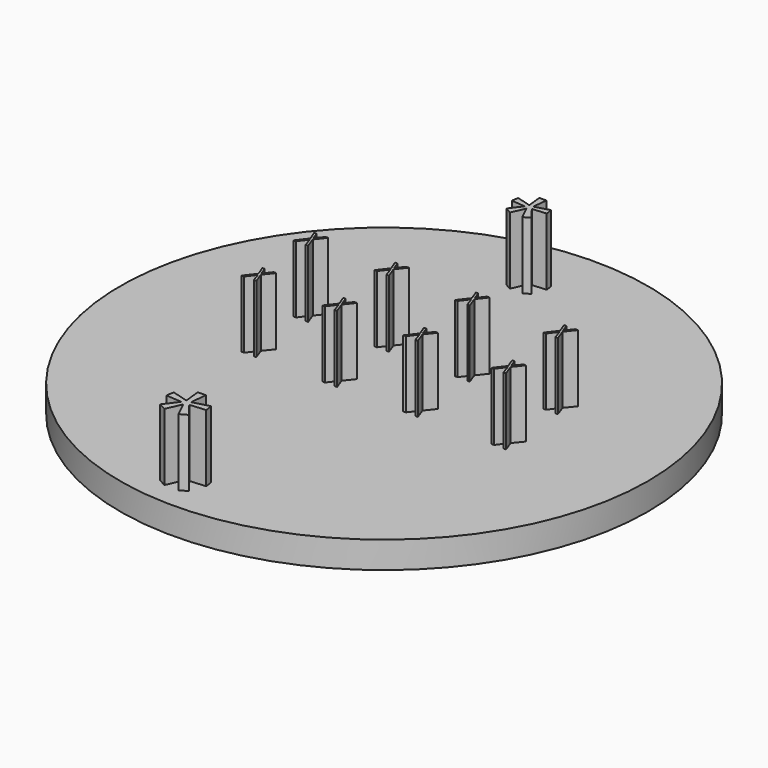
from build123d import *

# Parameters (mm, degrees)
F0_R         = 62.488790567
F5_DEPTH     = 3.175
F1_TEXT_SIZE = 17.7966750411
F6_DEPTH     = 19.05
F2_TEXT_SIZE = 20.2513920764
F7_DEPTH     = 19.05
F3_TEXT_SIZE = 6.6943401199
F8_DEPTH     = 19.05
F4_TEXT_SIZE = 6.6943401199
F9_DEPTH     = 19.05


# Not quite as in the source:
# - the program builds the solid bodies; features that only make, move or delete a surface that nothing else refers to are left out
# - Text() gives the source's letters only with a copy of the font that has no kerning and outlines rounded to 1/6400 em; it was checked with that copy


with BuildPart() as f5:
    # F0 (on Top) → F5 (new body, symmetric)
    with BuildSketch(Plane.XY):
        Circle(F0_R)
        Polygon((-25.9728055469, -3.9892201875), (-25.0638396775, -6.4995977325), (-25.6527324099, -6.4995977325), (-26.3493621787, -4.4044784731), (-27.9214861162, -6.4995977325), (-28.5292066802, -6.4995977325), (-26.5805261109, -3.9630704214), (-27.4403304201, -1.7204664812), (-26.8786334444, -1.7204664812), (-26.2144293856, -3.5614100142), (-24.7667783347, -1.7204664812), (-24.1590577707, -1.7204664812), align=None, mode=Mode.SUBTRACT)
        Polygon((-6.8426826636, -3.9892201875), (-5.9337167942, -6.4995977325), (-6.5226095266, -6.4995977325), (-7.2192392954, -4.4044784731), (-8.7913632329, -6.4995977325), (-9.3990837969, -6.4995977325), (-7.4504032276, -3.9630704214), (-8.3102075368, -1.7204664812), (-7.7485105611, -1.7204664812), (-7.0843065023, -3.5614100142), (-5.6366554514, -1.7204664812), (-5.0289348874, -1.7204664812), align=None, mode=Mode.SUBTRACT)
        Polygon((12.2874402197, -3.9892201875), (13.1964060891, -6.4995977325), (12.6075133567, -6.4995977325), (11.910883588, -4.4044784731), (10.3387596504, -6.4995977325), (9.7310390864, -6.4995977325), (11.6797196557, -3.9630704214), (10.8199153465, -1.7204664812), (11.3816123222, -1.7204664812), (12.045816381, -3.5614100142), (13.4934674319, -1.7204664812), (14.1011879959, -1.7204664812), align=None, mode=Mode.SUBTRACT)
        Polygon((33.1570455435, -3.9892201875), (34.066011413, -6.4995977325), (33.4771186805, -6.4995977325), (32.7804889118, -4.4044784731), (31.2083649743, -6.4995977325), (30.6006444103, -6.4995977325), (32.5493249795, -3.9630704214), (31.6895206704, -1.7204664812), (32.2512176461, -1.7204664812), (32.9154217048, -3.5614100142), (34.3630727558, -1.7204664812), (34.9707933198, -1.7204664812), align=None, mode=Mode.SUBTRACT)
    extrude(amount=F5_DEPTH, both=True)

    # F2 (on Top) → F7 (join)
    with BuildSketch(Plane.XY):
        with Locations((-10.2649243587, -63.4052827954)):
            Text('*', F2_TEXT_SIZE, font='Open Sans', text_align=(TextAlign.LEFT, TextAlign.BOTTOM))
    extrude(amount=F7_DEPTH)


with BuildPart() as f6:
    # F1 (on Top) → F6 (new body)
    with BuildSketch(Plane.XY):
        with Locations((-9.0206896615, 38.6617516757)):
            Text('*', F1_TEXT_SIZE, font='Open Sans', text_align=(TextAlign.LEFT, TextAlign.BOTTOM))
    extrude(amount=F6_DEPTH)


with BuildPart() as f8:
    # F3 (on Top) → F8 (new body)
    with BuildSketch(Plane.XY):
        with Locations((-28.189259721, -6.4995977325)):
            Text('X         X         X          X', F3_TEXT_SIZE, font='Open Sans', font_style=FontStyle.ITALIC, text_align=(TextAlign.LEFT, TextAlign.BOTTOM))
    extrude(amount=F8_DEPTH)


with BuildPart() as f9:
    # F4 (on Top) → F9 (new body)
    with BuildSketch(Plane.XY):
        with Locations((-29.5147999656, 10.5115697491)):
            Text('X         X         X          X', F4_TEXT_SIZE, font='Open Sans', font_style=FontStyle.ITALIC, text_align=(TextAlign.LEFT, TextAlign.BOTTOM))
    extrude(amount=F9_DEPTH)


solid = Compound([f5.part, f6.part, f8.part, f9.part])
